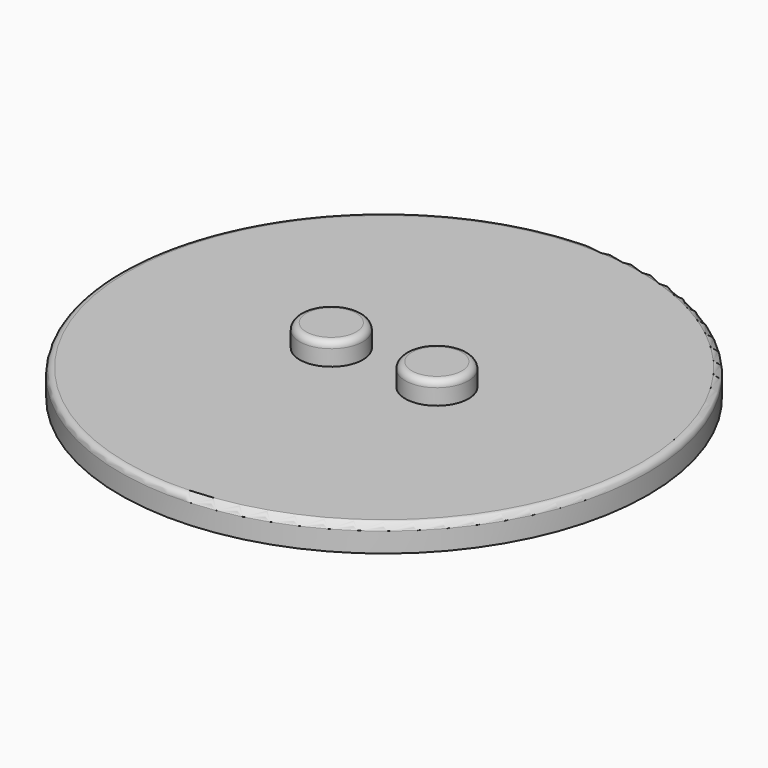
from build123d import *

# Parameters (mm, degrees)
F0_R     = 2.4
F1_DEPTH = 1.7
F0_R_2   = 20
F2_DEPTH = 2
F3_R     = 0.5
F4_DEPTH = 2


with BuildPart() as f1:
    # F0 (on Top) → F1 (new body)
    with BuildSketch(Plane.XY):
        with Locations((-4, 0)):
            Circle(F0_R)
    extrude(amount=F1_DEPTH)



with BuildPart() as f1b:
    # F0 (on Top) → F1, piece 2 (new body)
    with BuildSketch(Plane.XY):
        with Locations((4, 0)):
            Circle(F0_R)
    extrude(amount=F1_DEPTH)


with BuildPart() as f1_1:
    add(f1.part)

    add(f1b.part)  # F2 merges F1b
    # F0 (on Top) → F2 (join)
    with BuildSketch(Plane.XY):
        Circle(F0_R_2)
        with Locations((-4, 0)):
            Circle(F0_R, mode=Mode.SUBTRACT)
        with Locations((4, 0)):
            Circle(F0_R, mode=Mode.SUBTRACT)
    extrude(amount=-F2_DEPTH)

    # F3
    f3_edges = [f1_1.edges().sort_by_distance(p)[0] for p in [
        (-6.4, 0, 1.7),
        (1.6, 0, 1.7),
        (-20, 0, 0),
    ]]
    fillet(f3_edges, radius=F3_R)

    # F4 (add): faces of the model
    f4_faces = [f1_1.faces().sort_by_distance(p)[0] for p in [
        (-4, 0, 0),
        (4, 0, 0),
    ]]
    extrude(f4_faces, amount=F4_DEPTH)


solid = f1_1.part
